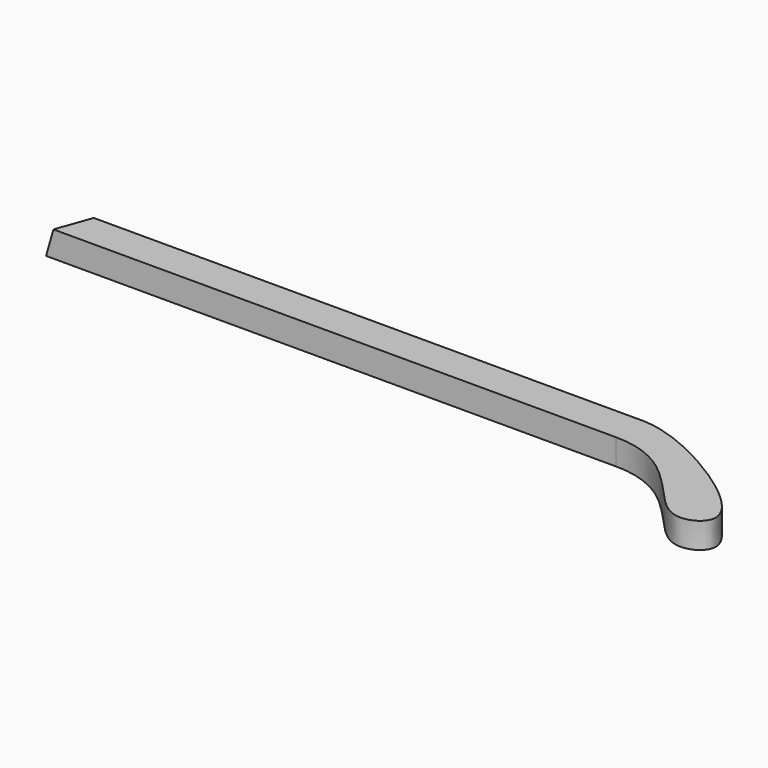
from build123d import *

# Parameters (mm, degrees)
F1_DEPTH = 3
F2_SIZE2 = 0.803838
F2_SIZE  = 2.99999


# Not quite as in the source:
# - a fillet or chamfer is up to 0.001 mm smaller than in the source, because OpenCascade refuses the exact size


with BuildPart() as f1:
    # F0 (on Top) → F1 (new body)
    with BuildSketch(Plane.XY):
        with BuildLine():
            Line((-34.3107653813, 4.0617076386), (-34.3107653813, 0))
            Line((-34.3107653813, 0), (30.6892346187, 0))
            add(Edge.make_bspline(
                [(30.6892346187, 0), (38.175922445, 0), (42.1268090367, -10.953828662), (50.634781902, -6.6086722293), (39.010439615, 1.9139667015), (32.7962212222, 3.9954856778), (30.6892346187, 4.0617076386)],
                knots=[0, 0, 0, 0, 0.322048395, 0.4820718301, 0.7572852316, 1, 1, 1, 1], degree=3))
            Line((30.6892346187, 4.0617076386), (-34.3107653813, 4.0617076386))
        make_face()
        Polygon((-35.7737392187, 0), (-34.3107653813, 0), (-34.3107653813, 4.0617076386), align=None)
    extrude(amount=F1_DEPTH)

    # F2 (size 3 and 0.8038475773 in the source; OpenCascade refuses exactly that, so slightly less here)
    f2_edges = [f1.edges().sort_by_distance(p)[0] for p in [
        (-35.042252, 2.030854, 3),
    ]]
    f2_side = f1.faces().sort_by_distance((-35.042252, 2.030854, 1.5))[0]
    chamfer(f2_edges, length=F2_SIZE, length2=F2_SIZE2, reference=f2_side)


solid = f1.part
